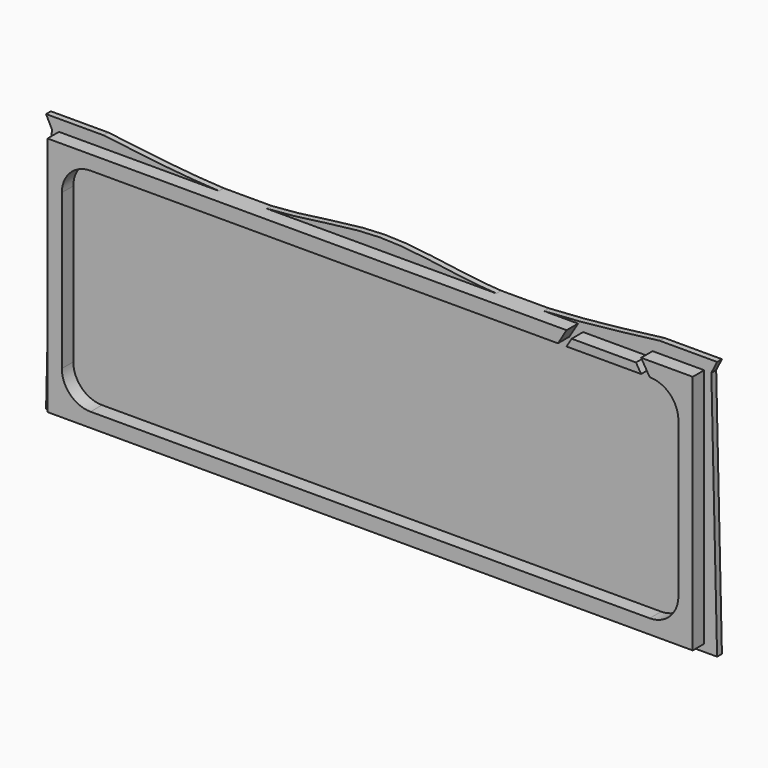
from build123d import *

# Parameters (mm, degrees)
F0_W     = 584.2
F0_H     = 219.71
F1_DEPTH = 5.334
F2_W     = 571.5
F2_H     = 213.36
F2_W_2   = 546.1
F2_H_2   = 187.96
F3_DEPTH = 12.7
F4_R     = 25.4
F6_DEPTH = 12.7
F8_DEPTH = 5.334


# Not quite as in the source:
# - a feature names something its author has since deleted; it is built from what else it names


with BuildPart() as f1:
    # F0 (on Front) → F1 (new body)
    with BuildSketch(Plane.XZ):
        with Locations((-292.1, 109.855)):
            Rectangle(F0_W, F0_H)
    extrude(amount=F1_DEPTH)

    # F2 (on face) → F3 (join)
    with BuildSketch(Plane.XZ.offset(5.334)):
        with Locations((-292.1, 113.03)):
            Rectangle(F2_W, F2_H)
        with Locations((-292.1, 113.03)):
            Rectangle(F2_W_2, F2_H_2, mode=Mode.SUBTRACT)
    extrude(amount=F3_DEPTH)

    # F4
    f4_edges = [f1.edges().sort_by_distance(p)[0] for p in [
        (-565.15, -11.684, 207.01),
        (-19.05, -11.684, 207.01),
        (-19.05, -11.684, 19.05),
        (-565.15, -11.684, 19.05),
    ]]
    fillet(f4_edges, radius=F4_R)

    # F5 (on face) → F6 (cut)
    with BuildSketch(Plane.XZ.offset(18.034)):
        Polygon((-118.11, 219.71), (-125.73, 207.01), (-118.11, 207.01), (-113.5820166854, 214.5566388576), (-110.49, 219.71), align=None)
        Polygon((-56.5979833146, 214.5566388576), (-52.07, 207.01), (-44.45, 207.01), (-52.07, 219.71), (-59.69, 219.71), align=None)
        Polygon((-59.69, 219.71), (-110.49, 219.71), (-113.5820166854, 214.5566388576), (-56.5979833146, 214.5566388576), align=None)
    extrude(amount=-F6_DEPTH, mode=Mode.SUBTRACT)

    # F7 (on face) → F8 (join)
    with BuildSketch(Plane(origin=(0, 0, 0), x_dir=(-1, 0, 0), z_dir=(0, 1, 0))):
        Polygon((-5.08, 0), (0, 0), (0, 219.71), align=None)
        Polygon((584.2, 219.71), (584.2, 0), (589.28, 0), align=None)
        with BuildLine():
            Line((-5.08, 229.87), (0, 219.71))
            Line((0, 219.71), (148.0852009026, 219.71))
            add(Edge.make_bspline(
                [(148.0852009026, 219.71), (115.3779899576, 221.1840971885), (80.5489949788, 225.5270485943), (45.72, 229.87)],
                knots=[0.812101374, 0.812101374, 0.812101374, 0.812101374, 1, 1, 1, 1], degree=3))
            Line((45.72, 229.87), (-5.08, 229.87))
        make_face()
        with BuildLine():
            Line((436.1147990974, 219.71), (584.2, 219.71))
            Line((584.2, 219.71), (589.28, 229.87))
            Line((589.28, 229.87), (538.48, 229.87))
            add(Edge.make_bspline(
                [(538.48, 229.87), (503.6510050212, 225.5270485943), (468.8220100424, 221.1840971885), (436.1147990974, 219.71)],
                knots=[0, 0, 0, 0, 0.187898626, 0.187898626, 0.187898626, 0.187898626], degree=3))
        make_face()
        with BuildLine():
            add(Edge.make_bspline(
                [(292.1, 229.87), (259.7414000619, 229.87), (227.3828001238, 221.731425099), (190.5, 219.71)],
                knots=[0.5, 0.5, 0.5, 0.5, 0.7280781407, 0.7280781407, 0.7280781407, 0.7280781407], degree=3))
            Line((190.5, 219.71), (393.7, 219.71))
            add(Edge.make_bspline(
                [(393.7, 219.71), (356.8171998762, 221.731425099), (324.4585999381, 229.87), (292.1, 229.87)],
                knots=[0.2719218593, 0.2719218593, 0.2719218593, 0.2719218593, 0.5, 0.5, 0.5, 0.5], degree=3))
        make_face()
    extrude(amount=-F8_DEPTH)


solid = f1.part
